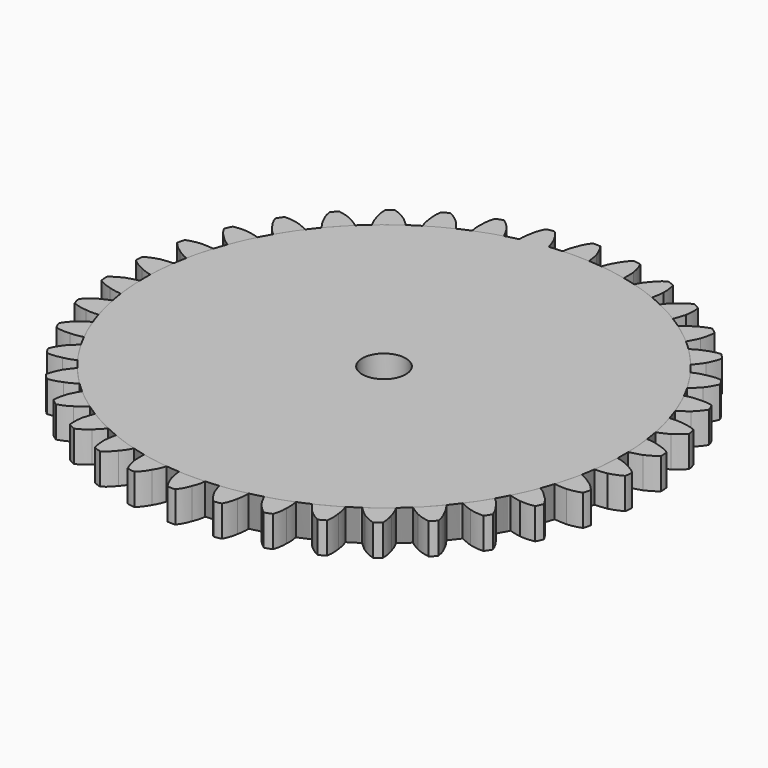
from build123d import *

# Parameters (mm, degrees)
F1_DEPTH = 5
F2_COUNT = 38
F3_R     = 3.5
F4_DEPTH = 12.5


with BuildPart() as f1:
    # F0 (on Top) → F1 (new body)
    with BuildSketch(Plane.XY):
        with BuildLine():
            ThreePointArc((-2.0174925217, 38.4471029328), (-26.500722046, -27.9277949549), (38.5, 0))
            ThreePointArc((38.5, 0), (27.9976842724, 26.426874113), (2.2205363437, 38.435910531))
            ThreePointArc((2.2205363437, 38.435910531), (0.1016760339, 38.4998657398), (-2.0174925217, 38.4471029328))
        make_face()
        with BuildLine():
            ThreePointArc((-2.0174925217, 38.4471029328), (0.1016760339, 38.4998657398), (2.2205363437, 38.435910531))
            ThreePointArc((2.2205363437, 38.435910531), (2.0710744369, 39.4233012517), (1.8625809871, 40.3999331058))
            Line((1.8625809871, 40.3999331058), (1.8525913839, 40.411282727))
            ThreePointArc((1.8525913839, 40.411282727), (1.4120282102, 41.4696953952), (0.8281605869, 42.4563219125))
            ThreePointArc((0.8281605869, 42.4563219125), (0.2001712308, 42.495206357), (-0.4278283139, 42.4564868122))
            ThreePointArc((-0.4278283139, 42.4564868122), (-1.0554145061, 41.4851608418), (-1.4990034031, 40.4171873122))
            ThreePointArc((-1.4990034031, 40.4171873122), (-1.8339404363, 39.4520659566), (-2.0174925217, 38.4471029328))
        make_face()
    extrude(amount=F1_DEPTH)


with BuildPart() as f2_1:
    # F2: instance of F1
    add(f1.part.rotate(Axis((0, 0, 0), (0, 0, -1)), 1 * 360 / F2_COUNT))


with BuildPart() as f2_2:
    # F2: instance of F1
    add(f1.part.rotate(Axis((0, 0, 0), (0, 0, -1)), 2 * 360 / F2_COUNT))


with BuildPart() as f2_3:
    # F2: instance of F1
    add(f1.part.rotate(Axis((0, 0, 0), (0, 0, -1)), 3 * 360 / F2_COUNT))


with BuildPart() as f2_4:
    # F2: instance of F1
    add(f1.part.rotate(Axis((0, 0, 0), (0, 0, -1)), 4 * 360 / F2_COUNT))


with BuildPart() as f2_5:
    # F2: instance of F1
    add(f1.part.rotate(Axis((0, 0, 0), (0, 0, -1)), 5 * 360 / F2_COUNT))


with BuildPart() as f2_6:
    # F2: instance of F1
    add(f1.part.rotate(Axis((0, 0, 0), (0, 0, -1)), 6 * 360 / F2_COUNT))


with BuildPart() as f2_7:
    # F2: instance of F1
    add(f1.part.rotate(Axis((0, 0, 0), (0, 0, -1)), 7 * 360 / F2_COUNT))


with BuildPart() as f2_8:
    # F2: instance of F1
    add(f1.part.rotate(Axis((0, 0, 0), (0, 0, -1)), 8 * 360 / F2_COUNT))


with BuildPart() as f2_9:
    # F2: instance of F1
    add(f1.part.rotate(Axis((0, 0, 0), (0, 0, -1)), 9 * 360 / F2_COUNT))


with BuildPart() as f2_10:
    # F2: instance of F1
    add(f1.part.rotate(Axis((0, 0, 0), (0, 0, -1)), 10 * 360 / F2_COUNT))


with BuildPart() as f2_11:
    # F2: instance of F1
    add(f1.part.rotate(Axis((0, 0, 0), (0, 0, -1)), 11 * 360 / F2_COUNT))


with BuildPart() as f2_12:
    # F2: instance of F1
    add(f1.part.rotate(Axis((0, 0, 0), (0, 0, -1)), 12 * 360 / F2_COUNT))


with BuildPart() as f2_13:
    # F2: instance of F1
    add(f1.part.rotate(Axis((0, 0, 0), (0, 0, -1)), 13 * 360 / F2_COUNT))


with BuildPart() as f2_14:
    # F2: instance of F1
    add(f1.part.rotate(Axis((0, 0, 0), (0, 0, -1)), 14 * 360 / F2_COUNT))


with BuildPart() as f2_15:
    # F2: instance of F1
    add(f1.part.rotate(Axis((0, 0, 0), (0, 0, -1)), 15 * 360 / F2_COUNT))


with BuildPart() as f2_16:
    # F2: instance of F1
    add(f1.part.rotate(Axis((0, 0, 0), (0, 0, -1)), 16 * 360 / F2_COUNT))


with BuildPart() as f2_17:
    # F2: instance of F1
    add(f1.part.rotate(Axis((0, 0, 0), (0, 0, -1)), 17 * 360 / F2_COUNT))


with BuildPart() as f2_18:
    # F2: instance of F1
    add(f1.part.rotate(Axis((0, 0, 0), (0, 0, -1)), 18 * 360 / F2_COUNT))


with BuildPart() as f2_19:
    # F2: instance of F1
    add(f1.part.rotate(Axis((0, 0, 0), (0, 0, -1)), 19 * 360 / F2_COUNT))


with BuildPart() as f2_20:
    # F2: instance of F1
    add(f1.part.rotate(Axis((0, 0, 0), (0, 0, -1)), 20 * 360 / F2_COUNT))


with BuildPart() as f2_21:
    # F2: instance of F1
    add(f1.part.rotate(Axis((0, 0, 0), (0, 0, -1)), 21 * 360 / F2_COUNT))


with BuildPart() as f2_22:
    # F2: instance of F1
    add(f1.part.rotate(Axis((0, 0, 0), (0, 0, -1)), 22 * 360 / F2_COUNT))


with BuildPart() as f2_23:
    # F2: instance of F1
    add(f1.part.rotate(Axis((0, 0, 0), (0, 0, -1)), 23 * 360 / F2_COUNT))


with BuildPart() as f2_24:
    # F2: instance of F1
    add(f1.part.rotate(Axis((0, 0, 0), (0, 0, -1)), 24 * 360 / F2_COUNT))


with BuildPart() as f2_25:
    # F2: instance of F1
    add(f1.part.rotate(Axis((0, 0, 0), (0, 0, -1)), 25 * 360 / F2_COUNT))


with BuildPart() as f2_26:
    # F2: instance of F1
    add(f1.part.rotate(Axis((0, 0, 0), (0, 0, -1)), 26 * 360 / F2_COUNT))


with BuildPart() as f2_27:
    # F2: instance of F1
    add(f1.part.rotate(Axis((0, 0, 0), (0, 0, -1)), 27 * 360 / F2_COUNT))


with BuildPart() as f2_28:
    # F2: instance of F1
    add(f1.part.rotate(Axis((0, 0, 0), (0, 0, -1)), 28 * 360 / F2_COUNT))


with BuildPart() as f2_29:
    # F2: instance of F1
    add(f1.part.rotate(Axis((0, 0, 0), (0, 0, -1)), 29 * 360 / F2_COUNT))


with BuildPart() as f2_30:
    # F2: instance of F1
    add(f1.part.rotate(Axis((0, 0, 0), (0, 0, -1)), 30 * 360 / F2_COUNT))


with BuildPart() as f2_31:
    # F2: instance of F1
    add(f1.part.rotate(Axis((0, 0, 0), (0, 0, -1)), 31 * 360 / F2_COUNT))


with BuildPart() as f2_32:
    # F2: instance of F1
    add(f1.part.rotate(Axis((0, 0, 0), (0, 0, -1)), 32 * 360 / F2_COUNT))


with BuildPart() as f2_33:
    # F2: instance of F1
    add(f1.part.rotate(Axis((0, 0, 0), (0, 0, -1)), 33 * 360 / F2_COUNT))


with BuildPart() as f2_34:
    # F2: instance of F1
    add(f1.part.rotate(Axis((0, 0, 0), (0, 0, -1)), 34 * 360 / F2_COUNT))


with BuildPart() as f2_35:
    # F2: instance of F1
    add(f1.part.rotate(Axis((0, 0, 0), (0, 0, -1)), 35 * 360 / F2_COUNT))


with BuildPart() as f2_36:
    # F2: instance of F1
    add(f1.part.rotate(Axis((0, 0, 0), (0, 0, -1)), 36 * 360 / F2_COUNT))


with BuildPart() as f2_37:
    # F2: instance of F1
    add(f1.part.rotate(Axis((0, 0, 0), (0, 0, -1)), 37 * 360 / F2_COUNT))


with BuildPart() as f4_tool:
    # F3 (on face) → F4 (new body, symmetric)
    with BuildSketch(Plane.XY.offset(5)):
        Circle(F3_R)
    extrude(amount=F4_DEPTH, both=True)


with BuildPart() as f1_1:
    add(f1.part)

    # F4: cut by f4_tool
    add(f4_tool.part, mode=Mode.SUBTRACT)


with BuildPart() as f2_1_1:
    add(f2_1.part)

    # F4: cut by f4_tool
    add(f4_tool.part, mode=Mode.SUBTRACT)


with BuildPart() as f2_2_1:
    add(f2_2.part)

    # F4: cut by f4_tool
    add(f4_tool.part, mode=Mode.SUBTRACT)


with BuildPart() as f2_3_1:
    add(f2_3.part)

    # F4: cut by f4_tool
    add(f4_tool.part, mode=Mode.SUBTRACT)


with BuildPart() as f2_4_1:
    add(f2_4.part)

    # F4: cut by f4_tool
    add(f4_tool.part, mode=Mode.SUBTRACT)


with BuildPart() as f2_5_1:
    add(f2_5.part)

    # F4: cut by f4_tool
    add(f4_tool.part, mode=Mode.SUBTRACT)


with BuildPart() as f2_6_1:
    add(f2_6.part)

    # F4: cut by f4_tool
    add(f4_tool.part, mode=Mode.SUBTRACT)


with BuildPart() as f2_7_1:
    add(f2_7.part)

    # F4: cut by f4_tool
    add(f4_tool.part, mode=Mode.SUBTRACT)


with BuildPart() as f2_8_1:
    add(f2_8.part)

    # F4: cut by f4_tool
    add(f4_tool.part, mode=Mode.SUBTRACT)


with BuildPart() as f2_9_1:
    add(f2_9.part)

    # F4: cut by f4_tool
    add(f4_tool.part, mode=Mode.SUBTRACT)


with BuildPart() as f2_10_1:
    add(f2_10.part)

    # F4: cut by f4_tool
    add(f4_tool.part, mode=Mode.SUBTRACT)


with BuildPart() as f2_11_1:
    add(f2_11.part)

    # F4: cut by f4_tool
    add(f4_tool.part, mode=Mode.SUBTRACT)


with BuildPart() as f2_12_1:
    add(f2_12.part)

    # F4: cut by f4_tool
    add(f4_tool.part, mode=Mode.SUBTRACT)


with BuildPart() as f2_13_1:
    add(f2_13.part)

    # F4: cut by f4_tool
    add(f4_tool.part, mode=Mode.SUBTRACT)


with BuildPart() as f2_14_1:
    add(f2_14.part)

    # F4: cut by f4_tool
    add(f4_tool.part, mode=Mode.SUBTRACT)


with BuildPart() as f2_15_1:
    add(f2_15.part)

    # F4: cut by f4_tool
    add(f4_tool.part, mode=Mode.SUBTRACT)


with BuildPart() as f2_16_1:
    add(f2_16.part)

    # F4: cut by f4_tool
    add(f4_tool.part, mode=Mode.SUBTRACT)


with BuildPart() as f2_17_1:
    add(f2_17.part)

    # F4: cut by f4_tool
    add(f4_tool.part, mode=Mode.SUBTRACT)


with BuildPart() as f2_18_1:
    add(f2_18.part)

    # F4: cut by f4_tool
    add(f4_tool.part, mode=Mode.SUBTRACT)


with BuildPart() as f2_19_1:
    add(f2_19.part)

    # F4: cut by f4_tool
    add(f4_tool.part, mode=Mode.SUBTRACT)


with BuildPart() as f2_20_1:
    add(f2_20.part)

    # F4: cut by f4_tool
    add(f4_tool.part, mode=Mode.SUBTRACT)


with BuildPart() as f2_21_1:
    add(f2_21.part)

    # F4: cut by f4_tool
    add(f4_tool.part, mode=Mode.SUBTRACT)


with BuildPart() as f2_22_1:
    add(f2_22.part)

    # F4: cut by f4_tool
    add(f4_tool.part, mode=Mode.SUBTRACT)


with BuildPart() as f2_23_1:
    add(f2_23.part)

    # F4: cut by f4_tool
    add(f4_tool.part, mode=Mode.SUBTRACT)


with BuildPart() as f2_24_1:
    add(f2_24.part)

    # F4: cut by f4_tool
    add(f4_tool.part, mode=Mode.SUBTRACT)


with BuildPart() as f2_25_1:
    add(f2_25.part)

    # F4: cut by f4_tool
    add(f4_tool.part, mode=Mode.SUBTRACT)


with BuildPart() as f2_26_1:
    add(f2_26.part)

    # F4: cut by f4_tool
    add(f4_tool.part, mode=Mode.SUBTRACT)


with BuildPart() as f2_27_1:
    add(f2_27.part)

    # F4: cut by f4_tool
    add(f4_tool.part, mode=Mode.SUBTRACT)


with BuildPart() as f2_28_1:
    add(f2_28.part)

    # F4: cut by f4_tool
    add(f4_tool.part, mode=Mode.SUBTRACT)


with BuildPart() as f2_29_1:
    add(f2_29.part)

    # F4: cut by f4_tool
    add(f4_tool.part, mode=Mode.SUBTRACT)


with BuildPart() as f2_30_1:
    add(f2_30.part)

    # F4: cut by f4_tool
    add(f4_tool.part, mode=Mode.SUBTRACT)


with BuildPart() as f2_31_1:
    add(f2_31.part)

    # F4: cut by f4_tool
    add(f4_tool.part, mode=Mode.SUBTRACT)


with BuildPart() as f2_32_1:
    add(f2_32.part)

    # F4: cut by f4_tool
    add(f4_tool.part, mode=Mode.SUBTRACT)


with BuildPart() as f2_33_1:
    add(f2_33.part)

    # F4: cut by f4_tool
    add(f4_tool.part, mode=Mode.SUBTRACT)


with BuildPart() as f2_34_1:
    add(f2_34.part)

    # F4: cut by f4_tool
    add(f4_tool.part, mode=Mode.SUBTRACT)


with BuildPart() as f2_35_1:
    add(f2_35.part)

    # F4: cut by f4_tool
    add(f4_tool.part, mode=Mode.SUBTRACT)


with BuildPart() as f2_36_1:
    add(f2_36.part)

    # F4: cut by f4_tool
    add(f4_tool.part, mode=Mode.SUBTRACT)


with BuildPart() as f2_37_1:
    add(f2_37.part)

    # F4: cut by f4_tool
    add(f4_tool.part, mode=Mode.SUBTRACT)


solid = Compound([f1_1.part, f2_1_1.part, f2_2_1.part, f2_3_1.part, f2_4_1.part, f2_5_1.part, f2_6_1.part, f2_7_1.part, f2_8_1.part, f2_9_1.part, f2_10_1.part, f2_11_1.part, f2_12_1.part, f2_13_1.part, f2_14_1.part, f2_15_1.part, f2_16_1.part, f2_17_1.part, f2_18_1.part, f2_19_1.part, f2_20_1.part, f2_21_1.part, f2_22_1.part, f2_23_1.part, f2_24_1.part, f2_25_1.part, f2_26_1.part, f2_27_1.part, f2_28_1.part, f2_29_1.part, f2_30_1.part, f2_31_1.part, f2_32_1.part, f2_33_1.part, f2_34_1.part, f2_35_1.part, f2_36_1.part, f2_37_1.part])
